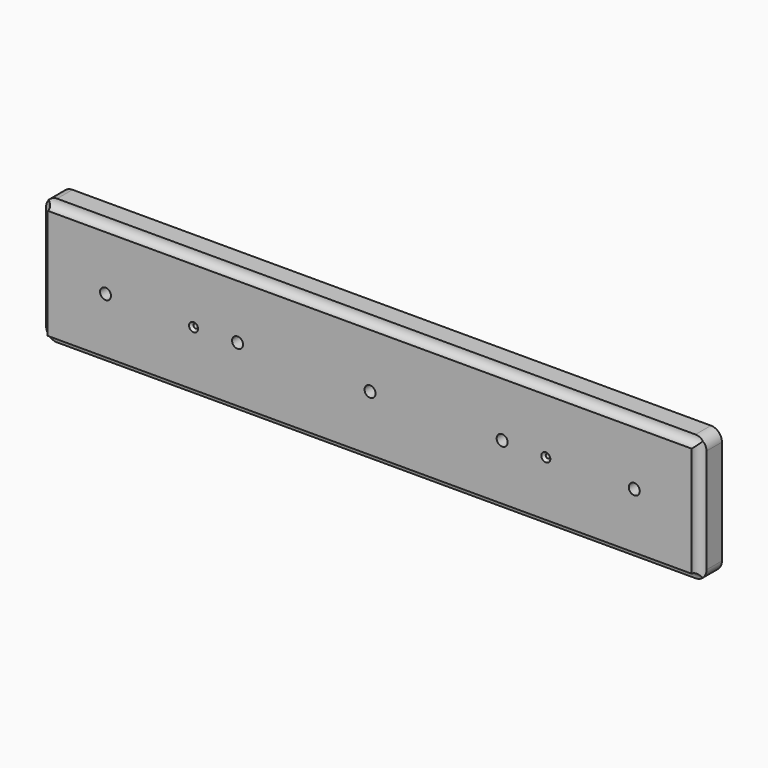
from build123d import *

# Parameters (mm, degrees)
F0_W            = 762
F0_H            = 146.05
F1_DEPTH        = 31.75
F2_R            = 9.525
F3_DEPTH        = 762.001
F4_R            = 9.525
F5_DEPTH        = 146.051
F6_R            = 9.525
F7_DEPTH        = 762.0010001
F8_R            = 9.5195259248
F9_DEPTH        = 146.0510001
F11_D           = 12.7
F11_DEPTH       = 19.05
F11_TIP         = 3.8154649308
F12_D           = 5.5
F12_CSINK_D     = 11.2
F12_CSINK_ANGLE = 90
F14_D           = 5.1054
F14_CSINK_D     = 10.4394
F14_CSINK_ANGLE = 82
F15_T1_DEPTH    = 85.725
F15_T3_DEPTH    = 85.7093782314


# Not quite as in the source:
# - a fillet or chamfer that OpenCascade refuses, or shapes differently, is made with other operations: its cross-section is extruded or revolved along the edge and cut away or added


with BuildPart() as f1:
    # F0 (on Front) → F1 (new body)
    with BuildSketch(Plane.XZ):
        Rectangle(F0_W, F0_H)
    extrude(amount=F1_DEPTH)

    # F2 (on face) → F3 (cut, through all)
    with BuildSketch(Plane(origin=(-381, 0, 0), x_dir=(0, -1, 0), z_dir=(-1, 0, 0))):
        with Locations((31.75, 73.025)):
            Circle(F2_R)
    extrude(amount=-F3_DEPTH, mode=Mode.SUBTRACT)

    # F4 (on face) → F5 (cut, through all)
    with BuildSketch(Plane.XY.offset(73.025)):
        with Locations((-380.995452404, -31.7343771458)):
            Circle(F4_R)
    extrude(amount=-F5_DEPTH, mode=Mode.SUBTRACT)

    # F6 (on face) → F7 (cut, through all)
    with BuildSketch(Plane.YZ.offset(381)):
        with Locations((-31.75, -73.025)):
            Circle(F6_R)
    extrude(amount=-F7_DEPTH, mode=Mode.SUBTRACT)

    # F8 (on face) → F9 (cut, through all)
    with BuildSketch(Plane(origin=(0, 0, -73.025), x_dir=(1, 0, 0), z_dir=(0, 0, -1))):
        with Locations((381.0260295868, 31.7688845098)):
            Circle(F8_R)
    extrude(amount=-F9_DEPTH, mode=Mode.SUBTRACT)

    # F11
    with Locations(Plane.XZ.offset(31.75)):
        with Locations((-304.7976701619, 0.8426916512), (-152.3976701619, 0.8426916512), (0.466863421, 0.8401229861), (152.866863421, 0.8401229861), (305.266863421, 0.8401229861)):
            Hole(F11_D / 2, depth=F11_DEPTH)
            with Locations((0, 0, -(F11_DEPTH + F11_TIP / 2))):  # 118° drill point
                Cone(0, F11_D / 2, F11_TIP, mode=Mode.SUBTRACT)

    # F12 (through all)
    with Locations(Plane(origin=(0, 0, 0), x_dir=(1, 0, 0), z_dir=(0, 1, 0))):
        with Locations((304.8, 0), (152.4, 0), (0, 0), (-152.4, 0), (-304.8, 0)):
            CounterSinkHole(F12_D / 2, F12_CSINK_D / 2, counter_sink_angle=F12_CSINK_ANGLE)

    # F14 (through all)
    with Locations(Plane.XZ.offset(31.75)):
        with Locations((-203.2, 0), (203.2, 0)):
            CounterSinkHole(F14_D / 2, F14_CSINK_D / 2, counter_sink_angle=F14_CSINK_ANGLE)

    # F15: fillet of radius 12.7 on 4 edges, made by hand

    # F15_s2 → F15_t1 (cut)
    with BuildSketch(Plane.XZ.offset(-31.75)):
        with BuildLine():
            ThreePointArc((368.3, 73.025), (377.2802561211, 69.3052561211), (381, 60.325))
            Line((381, 60.325), (381, 73.025))
            Line((381, 73.025), (368.3, 73.025))
        make_face()
        with BuildLine():
            ThreePointArc((381, -60.325), (377.2802561211, -69.3052561211), (368.3, -73.025))
            Line((368.3, -73.025), (381, -73.025))
            Line((381, -73.025), (381, -60.325))
        make_face()
    extrude(amount=F15_T1_DEPTH, mode=Mode.SUBTRACT)

    # F15_s4 → F15_t3 (cut)
    with BuildSketch(Plane.XZ.offset(-31.75)):
        with BuildLine():
            ThreePointArc((-368.3, 73.025), (-377.2802561211, 69.3052561211), (-381, 60.325))
            Line((-381, 60.325), (-381, 73.025))
            Line((-381, 73.025), (-368.3, 73.025))
        make_face()
        with BuildLine():
            ThreePointArc((-381, -60.325), (-377.2802561211, -69.3052561211), (-368.3, -73.025))
            Line((-368.3, -73.025), (-381, -73.025))
            Line((-381, -73.025), (-381, -60.325))
        make_face()
    extrude(amount=F15_T3_DEPTH, mode=Mode.SUBTRACT)


solid = f1.part
